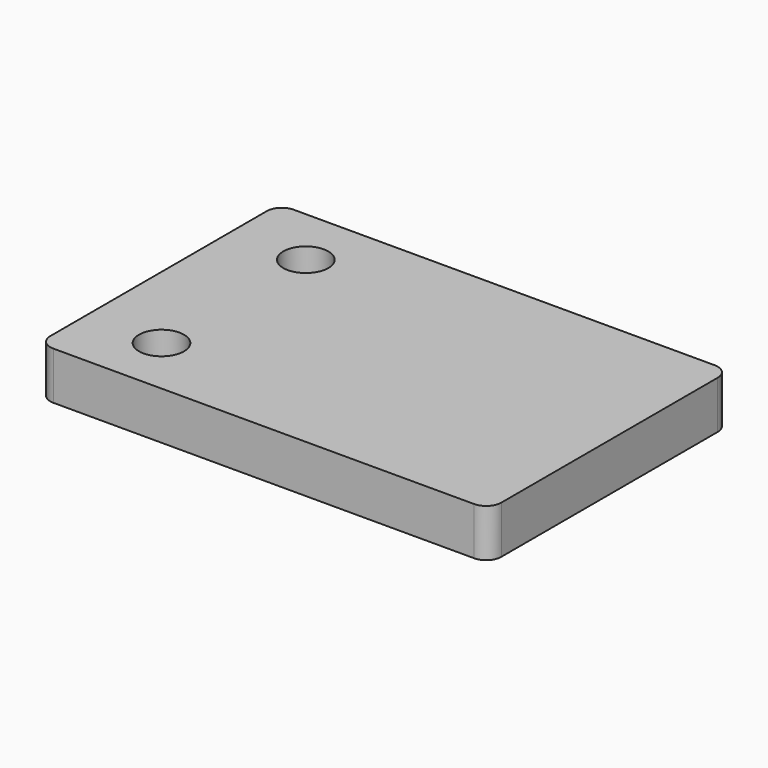
from build123d import *

# Parameters (mm, degrees)
F0_W     = 30
F0_H     = 20
F1_DEPTH = 3.175
F2_R     = 1.5
F3_DEPTH = 25
F4_R     = 1


# Not quite as in the source:
# - a length typed as a fraction of an inch, garbled in the dataset ("3 / 203.2 mm" for 3/8 in), is restored


with BuildPart() as f1:
    # F0 (on Top) → F1 (new body)
    with BuildSketch(Plane.XY):
        with Locations((15, 10)):
            Rectangle(F0_W, F0_H)
    extrude(amount=F1_DEPTH)

    # F2 (on face) → F3 (cut)
    with BuildSketch(Plane.XY.offset(3.175)):
        with Locations((5, 16)):
            Circle(F2_R)
        with Locations((5, 4)):
            Circle(F2_R)
    extrude(amount=-F3_DEPTH, mode=Mode.SUBTRACT)

    # F4
    f4_edges = [f1.edges().sort_by_distance(p)[0] for p in [
        (0, 20, 1.5875),
        (30, 20, 1.5875),
        (30, 0, 1.5875),
        (0, 0, 1.5875),
    ]]
    fillet(f4_edges, radius=F4_R)


solid = f1.part
